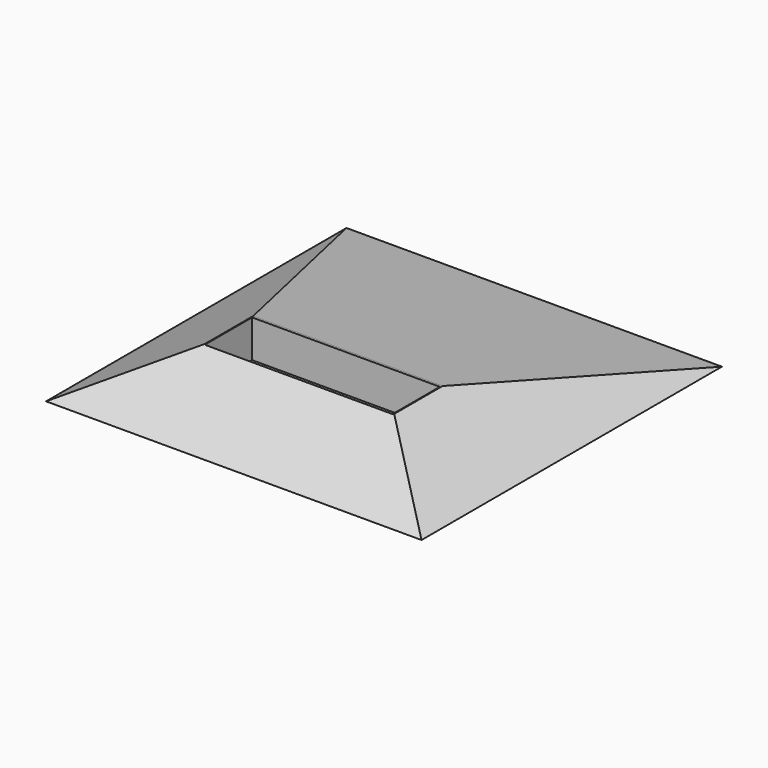
from build123d import *

# Parameters (mm, degrees)
F0_W        = 80
F0_H        = 80
F0_W_2      = 40
F0_H_2      = 12.5
F1_DEPTH    = 10.1
F2_T1_DEPTH = 170.5154722058
F3_SIZE2    = 19.822356
F3_SIZE     = 10.09999
F3_2_SIZE2  = 19.822356
F3_2_SIZE   = 10.09999
F4_SIZE2    = 49.643076
F4_SIZE     = 10.09999
F5_DEPTH    = 2.1


# Not quite as in the source:
# - a fillet or chamfer that OpenCascade refuses, or shapes differently, is made with other operations: its cross-section is extruded or revolved along the edge and cut away or added
# - a fillet or chamfer is up to 0.001 mm smaller than in the source, because OpenCascade refuses the exact size


with BuildPart() as f1:
    # F0 (on Top) → F1 (new body)
    with BuildSketch(Plane.XY):
        Rectangle(F0_W, F0_H)
        with Locations((0, -16.3821391761)):
            Rectangle(F0_W_2, F0_H_2, mode=Mode.SUBTRACT)
    extrude(amount=F1_DEPTH)

    # F2: chamfer of 10.1 x 17.4937131564 on 1 edges, made by hand

    # F2_s2 → F2_t1 (cut)
    with BuildSketch(Plane.YZ.offset(-85.2577361029)):
        Polygon((-40, 0), (-22.5062868436, 10.1), (-40, 10.1), align=None)
    extrude(amount=F2_T1_DEPTH, mode=Mode.SUBTRACT)

    # F3 (size 10.1 and 19.8223661056 in the source; OpenCascade refuses exactly that, so slightly less here)
    f3_edges = [f1.edges().sort_by_distance(p)[0] for p in [
        (-40, 8.746857, 10.1),
    ]]
    f3_side = f1.faces().sort_by_distance((-40, 4.194471, 4.843358))[0]
    chamfer(f3_edges, length=F3_SIZE, length2=F3_SIZE2, reference=f3_side)

    # F3#2 (size 10.1 and 19.8223661056 in the source; OpenCascade refuses exactly that, so slightly less here)
    f3_2_edges = [f1.edges().sort_by_distance(p)[0] for p in [
        (40, 8.746857, 10.1),
    ]]
    f3_2_side = f1.faces().sort_by_distance((40, 4.194471, 4.843358))[0]
    chamfer(f3_2_edges, length=F3_2_SIZE, length2=F3_2_SIZE2, reference=f3_2_side)

    # F4 (size 10.1 and 49.6430860138 in the source; OpenCascade refuses exactly that, so slightly less here)
    f4_edges = [f1.edges().sort_by_distance(p)[0] for p in [
        (0, 40, 10.1),
    ]]
    f4_side = f1.faces().sort_by_distance((0, 40, 4.495514))[0]
    chamfer(f4_edges, length=F4_SIZE, length2=F4_SIZE2, reference=f4_side)

    # F0 (on Top) → F5 (join)
    with BuildSketch(Plane.XY):
        with Locations((0, -16.3821391761)):
            Rectangle(F0_W_2, F0_H_2)
    extrude(amount=F5_DEPTH)


solid = f1.part
